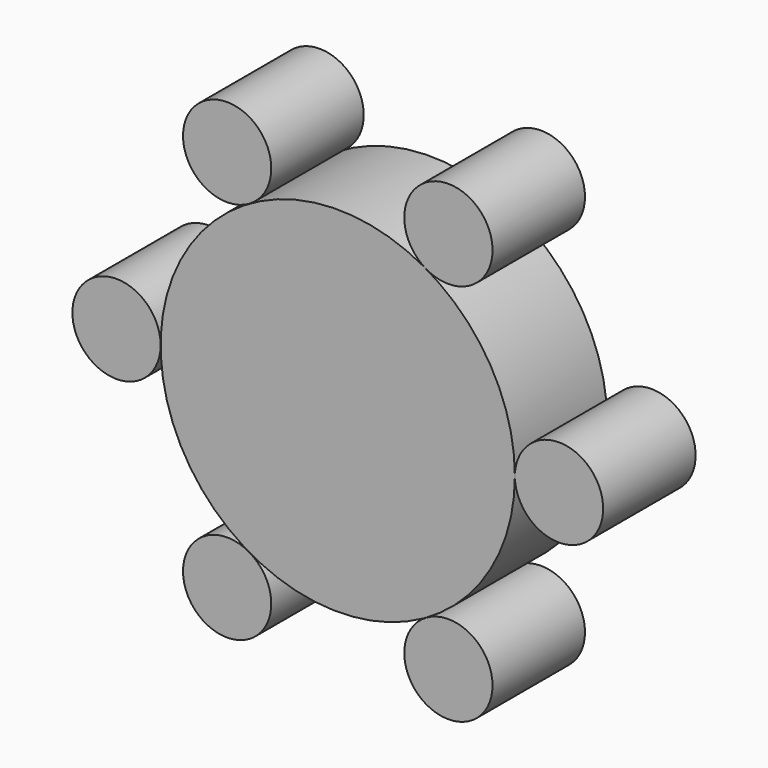
from build123d import *

# Parameters (mm, degrees)
F0_R     = 11.4557040809
F1_DEPTH = 30
F2_COUNT = 6


with BuildPart() as f1:
    # F0 (on Front) → F1 (new body)
    with BuildSketch(Plane.XZ):
        with Locations((-57.4294365942, 0)):
            Circle(F0_R)
    extrude(amount=F1_DEPTH)


with BuildPart() as f1b:
    # F0 (on Front) → F1, piece 2 (new body)
    with BuildSketch(Plane.XZ):
        with BuildLine():
            ThreePointArc((-45.9737325134, 0), (0, -45.9737325134), (45.9737325134, 0))
            ThreePointArc((45.9737325134, 0), (0, 45.9737325134), (-45.9737325134, 0))
        make_face()
    extrude(amount=F1_DEPTH)


with BuildPart() as f2_1:
    # F2: instance of F1
    add(f1.part.rotate(Axis((0, -30, 0), (0, 1, 0)), 1 * 360 / F2_COUNT))


with BuildPart() as f2_2:
    # F2: instance of F1
    add(f1.part.rotate(Axis((0, -30, 0), (0, 1, 0)), 2 * 360 / F2_COUNT))


with BuildPart() as f2_3:
    # F2: instance of F1
    add(f1.part.rotate(Axis((0, -30, 0), (0, 1, 0)), 3 * 360 / F2_COUNT))


with BuildPart() as f2_4:
    # F2: instance of F1
    add(f1.part.rotate(Axis((0, -30, 0), (0, 1, 0)), 4 * 360 / F2_COUNT))


with BuildPart() as f2_5:
    # F2: instance of F1
    add(f1.part.rotate(Axis((0, -30, 0), (0, 1, 0)), 5 * 360 / F2_COUNT))


solid = Compound([f1.part, f1b.part, f2_1.part, f2_2.part, f2_3.part, f2_4.part, f2_5.part])
